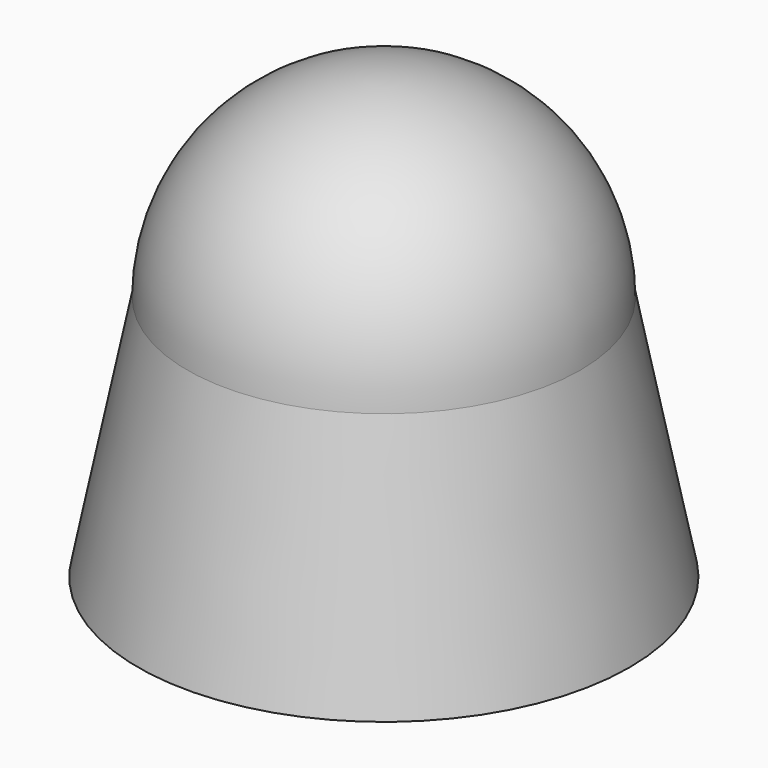
from build123d import *

# Parameters (mm, degrees)
F2_R     = 5
F2_R_2   = 4.7874181829
F3_DEPTH = 25
F4_DEPTH = 18
F2_R_3   = 13
F5_DEPTH = 6
F6_SIZE  = 3


# Not quite as in the source:
# - a feature names something its author has since deleted; it is built from what else it names


with BuildPart() as f1:
    # F0 (on Front) → F1 (revolve)
    with BuildSketch(Plane.XZ):
        with BuildLine():
            Line((0, 27), (0, 0))
            Line((0, 0), (15, 0))
            Line((15, 0), (12, 15))
            ThreePointArc((12, 15), (8.4852813742, 23.4852813742), (0, 27))
        make_face()
    revolve(axis=Axis((0, 0, 13.5), (0, 0, -1)))

    # F2 (on face) → F3 (cut)
    with BuildSketch(Plane(origin=(0, 0, 0), x_dir=(1, 0, 0), z_dir=(0, 0, -1))):
        Circle(F2_R)
        Circle(F2_R_2, mode=Mode.SUBTRACT)
        Circle(F2_R_2)
    extrude(amount=-F3_DEPTH, mode=Mode.SUBTRACT)

    # F2 (on face) → F4 (cut)
    with BuildSketch(Plane(origin=(0, 0, 0), x_dir=(1, 0, 0), z_dir=(0, 0, -1))):
        Polygon((9, -3.7279220614), (9, 3.7279220614), (3.7279220614, 9), (-3.7279220614, 9), (-9, 3.7279220614), (-9, -3.7279220614), (-3.7279220614, -9), (3.7279220614, -9), align=None)
        Circle(F2_R, mode=Mode.SUBTRACT)
    extrude(amount=-F4_DEPTH, mode=Mode.SUBTRACT)

    # F2 (on face) → F5 (cut)
    with BuildSketch(Plane(origin=(0, 0, 0), x_dir=(1, 0, 0), z_dir=(0, 0, -1))):
        Circle(F2_R_3)
        Polygon((3.7279220614, 9), (9, 3.7279220614), (9, -3.7279220614), (3.7279220614, -9), (-3.7279220614, -9), (-9, -3.7279220614), (-9, 3.7279220614), (-3.7279220614, 9), align=None, mode=Mode.SUBTRACT)
    extrude(amount=-F5_DEPTH, mode=Mode.SUBTRACT)

    # F6
    f6_edges = [f1.edges().sort_by_distance(p)[0] for p in [
        (-5, 0, 25),
        (-13, 0, 6),
        (0, 9, 18),
        (6.363961, 6.363961, 18),
        (9, 0, 18),
        (-6.363961, 6.363961, 18),
        (-9, 0, 18),
        (-6.363961, -6.363961, 18),
        (0, -9, 18),
        (6.363961, -6.363961, 18),
    ]]
    chamfer(f6_edges, length=F6_SIZE)


solid = f1.part
